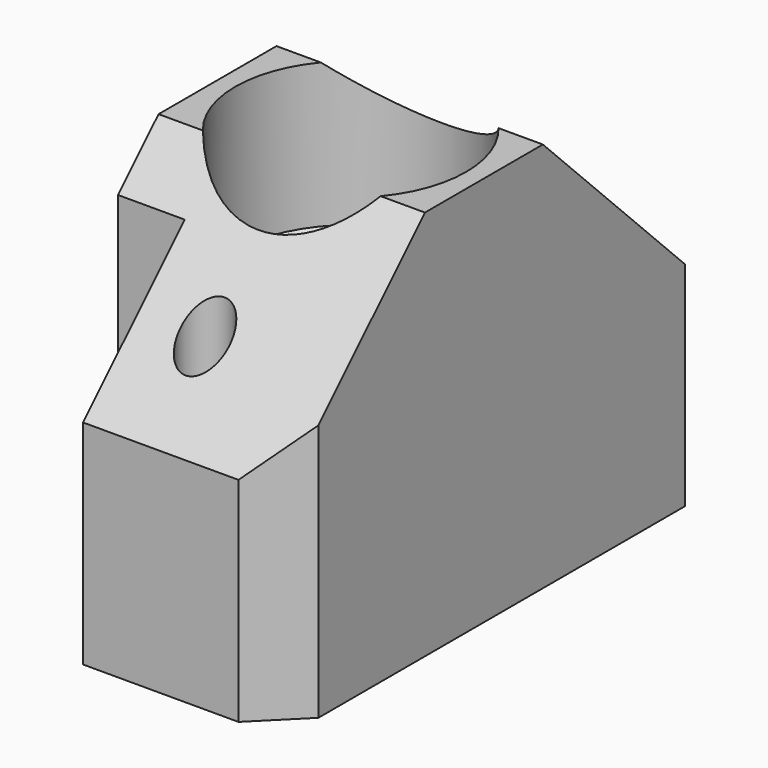
from build123d import *

# Parameters (mm, degrees)
F0_R        = 2.75
F0_R_2      = 13
F0_R_3      = 10.75
F1_DEPTH    = 30
F2_START    = 30
F2_DEPTH    = 14
F3_S5_R     = 13
F3_T6_DEPTH = 23
F4_SIZE     = 5
F5_T1_DEPTH = 117.8673195186
F5_T3_DEPTH = 120.3673195186


# Not quite as in the source:
# - a fillet or chamfer that OpenCascade refuses, or shapes differently, is made with other operations: its cross-section is extruded or revolved along the edge and cut away or added


with BuildPart() as f1:
    # F0 (on Top) → F1 (new body)
    with BuildSketch(Plane.XY):
        Polygon((0, 28.3), (0, 15), (-15, 15), (-15, -14), (-7.5, -14), (-7.5, -28.3), (0, -28.3), (15, -28.3), (15, 15), (15, 28.3), align=None)
        with Locations((0, -20.5)):
            Circle(F0_R, mode=Mode.SUBTRACT)
        Circle(F0_R_2, mode=Mode.SUBTRACT)
        Circle(F0_R_2)
        Circle(F0_R_3, mode=Mode.SUBTRACT)
    extrude(amount=F1_DEPTH)

    # F0 (on Top) → F2 (join)
    with BuildSketch(Plane.XY.offset(F2_START)):
        Polygon((0, 28.3), (0, 15), (-15, 15), (-15, -14), (-7.5, -14), (-7.5, -28.3), (0, -28.3), (15, -28.3), (15, 15), (15, 28.3), align=None)
        with Locations((0, -20.5)):
            Circle(F0_R, mode=Mode.SUBTRACT)
        Circle(F0_R_2, mode=Mode.SUBTRACT)
    extrude(amount=F2_DEPTH)

    # F3: chamfer of 4.5 on 1 edges, made by hand


with BuildPart() as f3_tool2:
    # F3_s3 → F3_t4 (revolve)
    with BuildSketch(Plane.XZ):
        Polygon((10.75, 25.5), (15.25, 30), (10.75, 30), align=None)
    revolve(axis=Axis((0, 0, 30), (0, 0, 1)))

    # F3_s5 → F3_t6 (intersect, symmetric)
    with BuildSketch(Plane.XY.offset(27.8)):
        Circle(F3_S5_R)
    extrude(amount=F3_T6_DEPTH, both=True, mode=Mode.INTERSECT)


with BuildPart() as f1_1:
    add(f1.part)

    # F3_t1: cut F3_tool2
    add(f3_tool2.part, mode=Mode.SUBTRACT)

    # F4
    f4_edges = [f1_1.edges().sort_by_distance(p)[0] for p in [
        (15, -28.3, 22),
    ]]
    chamfer(f4_edges, length=F4_SIZE)

    # F5: chamfer of 20 on 2 edges, made by hand

    # F5_s2 → F5_t1 (cut)
    with BuildSketch(Plane.YZ.offset(-51.4336597593)):
        Polygon((28.3, 24), (8.3, 44), (28.3, 44), align=None)
    extrude(amount=F5_T1_DEPTH, mode=Mode.SUBTRACT)

    # F5_s4 → F5_t3 (cut)
    with BuildSketch(Plane.YZ.offset(-58.9336597593)):
        Polygon((-28.3, 24), (-8.3, 44), (-28.3, 44), align=None)
    extrude(amount=F5_T3_DEPTH, mode=Mode.SUBTRACT)


solid = f1_1.part
